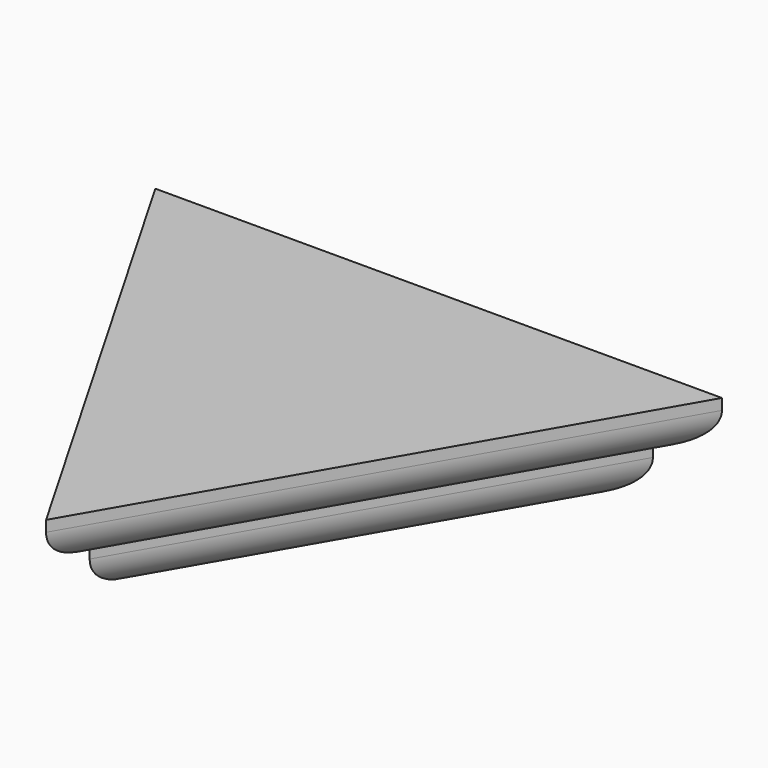
from build123d import *

# Parameters (mm, degrees)
F0_W         = 3
F0_H         = 20
F1_DEPTH     = 10
F2_DEPTH     = 5
F3_T1_DEPTH  = 70
F3_T3_DEPTH  = 79.20981353
F3_T5_DEPTH  = 70
F3_T7_DEPTH  = 70
F3_T9_DEPTH  = 79.20981353
F3_T11_DEPTH = 79.20981353


# Not quite as in the source:
# - a fillet or chamfer that OpenCascade refuses, or shapes differently, is made with other operations: its cross-section is extruded or revolved along the edge and cut away or added


with BuildPart() as f1:
    # F0 (on Top) → F1 (new body)
    with BuildSketch(Plane.XY):
        Polygon((25, 14.4337567297), (-25, 14.4337567297), (0, -28.8675134595), align=None)
        Rectangle(F0_W, F0_H, mode=Mode.SUBTRACT)
    extrude(amount=-F1_DEPTH)

    # F0 (on Top) → F2 (join)
    with BuildSketch(Plane.XY):
        Polygon((30, 17.3205080757), (-30, 17.3205080757), (0, -34.6410161514), align=None)
        Polygon((0, -28.8675134595), (-25, 14.4337567297), (25, 14.4337567297), align=None, mode=Mode.SUBTRACT)
        Rectangle(F0_W, F0_H)
    extrude(amount=-F2_DEPTH)

    # F3: fillet of radius 4 on 6 edges, made by hand

    # F3_s2 → F3_t1 (cut)
    with BuildSketch(Plane.YZ.offset(-35)):
        with BuildLine():
            ThreePointArc((14.4337567297, -6), (13.2621838545, -8.8284271247), (10.4337567297, -10))
            Line((10.4337567297, -10), (14.4337567297, -10))
            Line((14.4337567297, -10), (14.4337567297, -6))
        make_face()
    extrude(amount=F3_T1_DEPTH, mode=Mode.SUBTRACT)

    # F3_s4 → F3_t3 (cut)
    with BuildSketch(Plane.YZ.offset(-39.604906765)):
        with BuildLine():
            ThreePointArc((14.4337567297, -5), (16.5183975841, -3.5608487081), (17.3205080757, -1.158037294))
            Line((17.3205080757, -1.158037294), (17.3205080757, -5))
            Line((17.3205080757, -5), (14.4337567297, -5))
        make_face()
    extrude(amount=F3_T3_DEPTH, mode=Mode.SUBTRACT)

    # F3_s6 → F3_t5 (cut)
    with BuildSketch(Plane(origin=(-17.5, -30.3108891325, 0), x_dir=(0, 0, 1), z_dir=(0.5, 0.8660254038, 0))):
        with BuildLine():
            ThreePointArc((-10, 10.4337567297), (-8.8284271247, 13.2621838545), (-6, 14.4337567297))
            Line((-6, 14.4337567297), (-10, 14.4337567297))
            Line((-10, 14.4337567297), (-10, 10.4337567297))
        make_face()
    extrude(amount=F3_T5_DEPTH, mode=Mode.SUBTRACT)

    # F3_s8 → F3_t7 (cut)
    with BuildSketch(Plane(origin=(-17.5, 30.3108891325, 0), x_dir=(0, 0, 1), z_dir=(0.5, -0.8660254038, 0))):
        with BuildLine():
            ThreePointArc((-6, 14.4337567297), (-8.8284271247, 13.2621838545), (-10, 10.4337567297))
            Line((-10, 10.4337567297), (-10, 14.4337567297))
            Line((-10, 14.4337567297), (-6, 14.4337567297))
        make_face()
    extrude(amount=F3_T7_DEPTH, mode=Mode.SUBTRACT)

    # F3_s10 → F3_t9 (cut)
    with BuildSketch(Plane(origin=(-19.8024533825, -34.298855373, 0), x_dir=(0, 0, 1), z_dir=(0.5, 0.8660254038, 0))):
        with BuildLine():
            ThreePointArc((-5, 14.4337567297), (-3.5608487081, 16.5183975841), (-1.158037294, 17.3205080757))
            Line((-1.158037294, 17.3205080757), (-5, 17.3205080757))
            Line((-5, 17.3205080757), (-5, 14.4337567297))
        make_face()
    extrude(amount=F3_T9_DEPTH, mode=Mode.SUBTRACT)

    # F3_s12 → F3_t11 (cut)
    with BuildSketch(Plane(origin=(-19.8024533825, 34.298855373, 0), x_dir=(0, 0, 1), z_dir=(0.5, -0.8660254038, 0))):
        with BuildLine():
            ThreePointArc((-5, 14.4337567297), (-3.5608487081, 16.5183975841), (-1.158037294, 17.3205080757))
            Line((-1.158037294, 17.3205080757), (-5, 17.3205080757))
            Line((-5, 17.3205080757), (-5, 14.4337567297))
        make_face()
    extrude(amount=F3_T11_DEPTH, mode=Mode.SUBTRACT)


solid = f1.part
